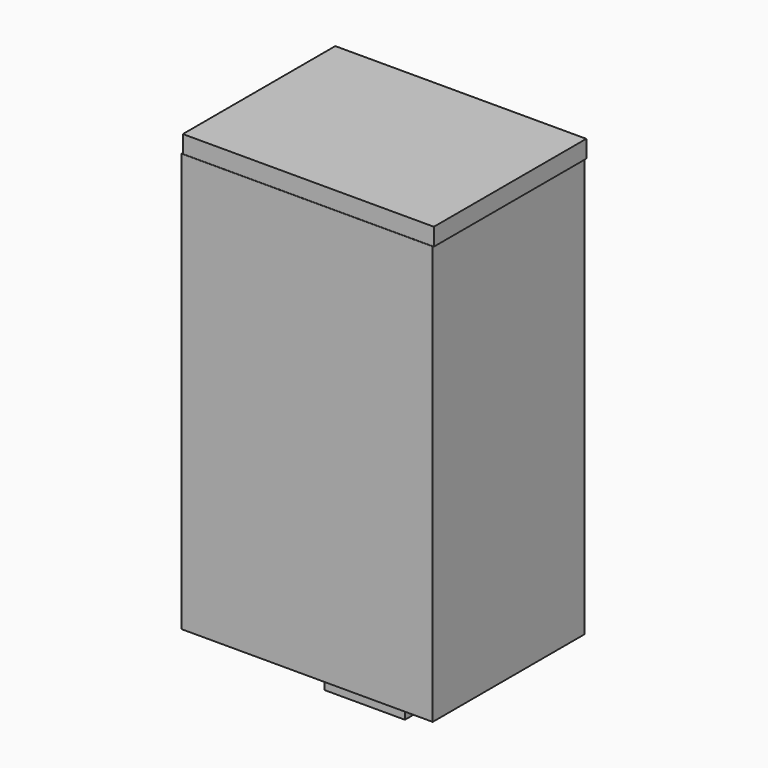
from build123d import *

# Parameters (mm, degrees)
F0_W      = 57.2311095893
F0_H      = 95.4614840448
F1_DEPTH  = 43.3
F2_T      = -2.5
F3_W      = 18.3139545843
F3_H      = 13.0486916751
F4_DEPTH  = 11.8
F5_T      = -2.5
F7_D      = 6.7564
F9_W      = 57.2428498417
F9_H      = 43.440643698
F10_DEPTH = 4


# Not quite as in the source:
# - a shell that OpenCascade refuses in one call is made with other operations: the cavity is built on its own and cut out


with BuildPart() as f1:
    # F0 (on Front) → F1 (new body)
    with BuildSketch(Plane.XZ):
        with Locations((1.2590847909, -3.6627892405)):
            Rectangle(F0_W, F0_H)
    extrude(amount=F1_DEPTH)

    # F2
    f2_openings = [f1.faces().sort_by_distance(p)[0] for p in [
        (1.259085, -21.65, 44.067953),
    ]]
    offset(amount=F2_T, openings=f2_openings)

    # F3 (on face) → F4 (join)
    with BuildSketch(Plane(origin=(0, 0, -51.3935312629), x_dir=(1, 0, 0), z_dir=(0, 0, -1))):
        with Locations((2.1747821011, 21.5188963339)):
            Rectangle(F3_W, F3_H)
    extrude(amount=F4_DEPTH)

    # F5: a shell. OpenCascade refuses it in one call, so the cavity is built on its own and cut out:
    # the body offset inwards by the wall thickness, plus a prism from it out through each open face.
    f5_core = offset(f1.part, amount=F5_T, kind=Kind.INTERSECTION, mode=Mode.PRIVATE)
    f5_exits = [f5_core.faces().sort_by_distance(p)[0] for p in [
        (2.174782, -21.518896, -60.693531),
    ]]
    add(f5_core, mode=Mode.SUBTRACT)
    extrude(f5_exits, amount=-F5_T, mode=Mode.SUBTRACT)

    # F7 (through all)
    with Locations(Plane(origin=(0, 0, -51.3935312629), x_dir=(1, 0, 0), z_dir=(0, 0, -1))):
        with Locations((1.8427748, 21.4465260506)):
            Hole(F7_D / 2)


with BuildPart() as f10:
    # F9 (on offset) → F10 (new body)
    with BuildSketch(Plane.XY.offset(44.2)):
        with Locations((1.6333451495, -21.720321849)):
            Rectangle(F9_W, F9_H)
    extrude(amount=F10_DEPTH)


solid = Compound([f1.part, f10.part])
